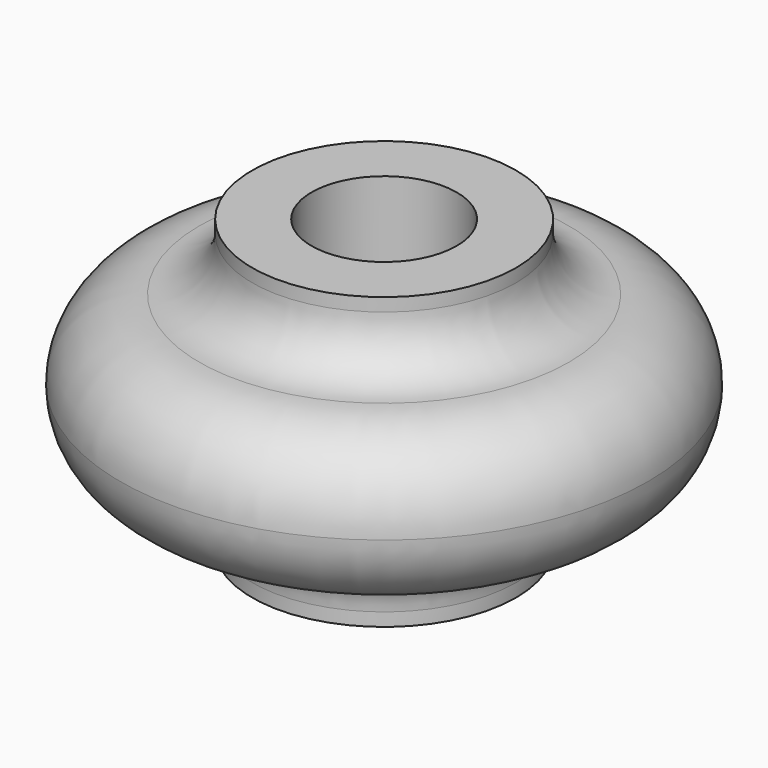
from build123d import *

# Parameters (mm, degrees)
F0_R     = 5
F0_R_2   = 2.75
F1_DEPTH = 5.5
F0_R_3   = 10
F2_DEPTH = 3
F3_R     = 2.99999
F4_R     = 2


# Not quite as in the source:
# - a fillet or chamfer is up to 0.001 mm smaller than in the source, because OpenCascade refuses the exact size


with BuildPart() as f1:
    # F0 (on Top) → F1 (new body, symmetric)
    with BuildSketch(Plane.XY):
        Circle(F0_R)
        Circle(F0_R_2, mode=Mode.SUBTRACT)
    extrude(amount=F1_DEPTH, both=True)

    # F0 (on Top) → F2 (join, symmetric)
    with BuildSketch(Plane.XY):
        Circle(F0_R_3)
        Circle(F0_R, mode=Mode.SUBTRACT)
    extrude(amount=F2_DEPTH, both=True)

    # F3 (radius 3 in the source; OpenCascade refuses exactly that, so slightly less here)
    f3_edges = [f1.edges().sort_by_distance(p)[0] for p in [
        (-10, 0, 3),
        (-10, 0, -3),
    ]]
    fillet(f3_edges, radius=F3_R)

    # F4
    f4_edges = [f1.edges().sort_by_distance(p)[0] for p in [
        (-5, 0, 3),
        (-5, 0, -3),
    ]]
    fillet(f4_edges, radius=F4_R)


solid = f1.part
